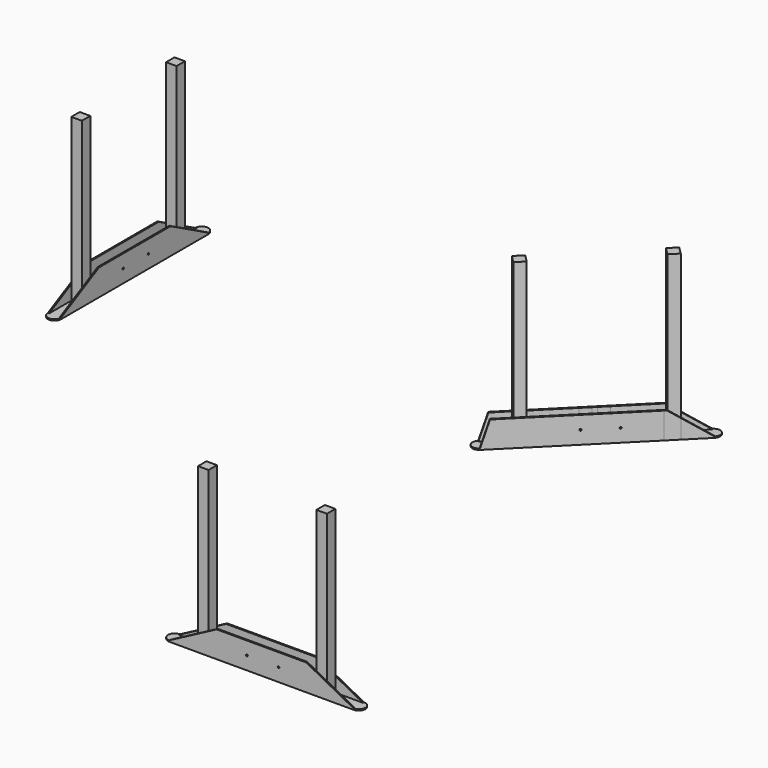
from build123d import *

# Parameters (mm, degrees)
F0_W           = 105
F0_H           = 40
F1_DEPTH       = 5
F0_W_2         = 40
F0_H_2         = 105
F2_DEPTH       = 620
F3_DEPTH       = 100
F4_T4_DEPTH    = 5
F4_T9_DEPTH    = 5
F4_T14_DEPTH   = 5
F4_T19_DEPTH   = 5
F4_2_T4_DEPTH  = 5
F4_2_T9_DEPTH  = 5
F4_2_T14_DEPTH = 5
F4_2_T19_DEPTH = 5
F6_T4_DEPTH    = 5
F6_T9_DEPTH    = 5
F7_SIZE2       = 94.99999
F7_SIZE        = 29.99999
F7_2_SIZE2     = 94.99999
F7_2_SIZE      = 29.99999
F10_R          = 3.25
F11_DEPTH      = 60
F12_R          = 3.25
F13_DEPTH      = 60
F14_R          = 3.25
F15_DEPTH      = 60


# Not quite as in the source:
# - a fillet or chamfer that OpenCascade refuses, or shapes differently, is made with other operations: its cross-section is extruded or revolved along the edge and cut away or added
# - two fillets or chamfers of one size are made in one step
# - a fillet or chamfer is up to 0.001 mm smaller than in the source, because OpenCascade refuses the exact size
# - a feature names something its author has since deleted; it is built from what else it names


with BuildPart() as f1:
    # F0 (on Top) → F1 (new body)
    with BuildSketch(Plane.XY):
        with BuildLine():
            ThreePointArc((811.153096903, -1265.8878414162), (836.153096903, -1240.8878414162), (811.153096903, -1215.8878414162))
            Line((811.153096903, -1215.8878414162), (811.153096903, -1220.8878414162))
            Line((811.153096903, -1220.8878414162), (811.153096903, -1260.8878414162))
            Line((811.153096903, -1260.8878414162), (811.153096903, -1265.8878414162))
        make_face()
        with Locations((758.653096903, -1240.8878414162)):
            Rectangle(F0_W, F0_H)
    extrude(amount=F1_DEPTH)



with BuildPart() as f1b:
    # F0 (on Top) → F1, piece 2 (new body)
    with BuildSketch(Plane.XY):
        with BuildLine():
            Line((111.153096903, -1220.8878414162), (111.153096903, -1215.8878414162))
            ThreePointArc((111.153096903, -1215.8878414162), (86.153096903, -1240.8878414162), (111.153096903, -1265.8878414162))
            Line((111.153096903, -1265.8878414162), (111.153096903, -1260.8878414162))
            Line((111.153096903, -1260.8878414162), (111.153096903, -1220.8878414162))
        make_face()
        with Locations((163.653096903, -1240.8878414162)):
            Rectangle(F0_W, F0_H)
    extrude(amount=F1_DEPTH)


with BuildPart() as f1c:
    # F0 (on Top) → F1, piece 3 (new body)
    with BuildSketch(Plane.XY):
        with BuildLine():
            Line((29.0142804433, 304.9314484107), (25.4787465374, 308.4669823167))
            ThreePointArc((25.4787465374, 308.4669823167), (25.4787465374, 273.1116432573), (60.8340855967, 273.1116432573))
            Line((60.8340855967, 273.1116432573), (57.2985516908, 276.6471771633))
            Line((57.2985516908, 276.6471771633), (29.0142804433, 304.9314484107))
        make_face()
        Polygon((99.724958562, 375.6421265294), (29.0142804433, 304.9314484107), (57.2985516908, 276.6471771633), (128.0092298094, 347.3578552819), align=None)
    extrude(amount=F1_DEPTH)



with BuildPart() as f1d:
    # F0 (on Top) → F1, piece 4 (new body)
    with BuildSketch(Plane.XY):
        with BuildLine():
            ThreePointArc((555.8088324273, 768.0863900879), (555.8088324273, 803.4417291473), (520.453493368, 803.4417291473))
            Line((520.453493368, 803.4417291473), (523.9890272739, 799.9061952413))
            Line((523.9890272739, 799.9061952413), (552.2732985214, 771.6219239939))
            Line((552.2732985214, 771.6219239939), (555.8088324273, 768.0863900879))
        make_face()
        Polygon((552.2732985214, 771.6219239939), (523.9890272739, 799.9061952413), (453.2783491552, 729.1955171227), (481.5626204027, 700.9112458752), align=None)
    extrude(amount=F1_DEPTH)


with BuildPart() as f1e:
    # F0 (on Top) → F1, piece 5 (new body)
    with BuildSketch(Plane.XY):
        with BuildLine():
            Line((-1479.9614127988, 152.1980424396), (-1484.9614127988, 152.1980424396))
            ThreePointArc((-1484.9614127988, 152.1980424396), (-1459.9614127988, 127.1980424396), (-1434.9614127988, 152.1980424396))
            Line((-1434.9614127988, 152.1980424396), (-1439.9614127988, 152.1980424396))
            Line((-1439.9614127988, 152.1980424396), (-1479.9614127988, 152.1980424396))
        make_face()
        Polygon((-1479.9614127988, 202.1980424396), (-1479.9614127988, 152.1980424396), (-1439.9614127988, 152.1980424396), (-1439.9614127988, 202.1980424396), (-1439.9614127988, 242.1980424396), (-1439.9614127988, 257.1980424396), (-1479.9614127988, 257.1980424396), (-1479.9614127988, 242.1980424396), align=None)
    extrude(amount=F1_DEPTH)



with BuildPart() as f1f:
    # F0 (on Top) → F1, piece 6 (new body)
    with BuildSketch(Plane.XY):
        with BuildLine():
            ThreePointArc((-1434.9614127988, 852.1980424396), (-1459.9614127988, 877.1980424396), (-1484.9614127988, 852.1980424396))
            Line((-1484.9614127988, 852.1980424396), (-1479.9614127988, 852.1980424396))
            Line((-1479.9614127988, 852.1980424396), (-1439.9614127988, 852.1980424396))
            Line((-1439.9614127988, 852.1980424396), (-1434.9614127988, 852.1980424396))
        make_face()
        with Locations((-1459.9614127988, 799.6980424396)):
            Rectangle(F0_W_2, F0_H_2)
    extrude(amount=F1_DEPTH)


with BuildPart() as f1g:
    # F0 (on Top) → F1, piece 7 (new body)
    with BuildSketch(Plane.XY):
        Polygon((331.153096903, -1220.8878414162), (256.153096903, -1220.8878414162), (256.153096903, -1260.8878414162), (331.153096903, -1260.8878414162), (421.153096903, -1260.8878414162), (511.153096903, -1260.8878414162), (591.153096903, -1260.8878414162), (666.153096903, -1260.8878414162), (666.153096903, -1220.8878414162), (591.153096903, -1220.8878414162), (511.153096903, -1220.8878414162), (421.153096903, -1220.8878414162), align=None)
    extrude(amount=F1_DEPTH)


with BuildPart() as f1h:
    # F0 (on Top) → F1, piece 8 (new body)
    with BuildSketch(Plane.XY):
        Polygon((-1439.9614127988, 707.1980424396), (-1479.9614127988, 707.1980424396), (-1479.9614127988, 542.1980424396), (-1479.9614127988, 502.1980424396), (-1479.9614127988, 297.1980424396), (-1439.9614127988, 297.1980424396), (-1439.9614127988, 502.1980424396), (-1439.9614127988, 542.1980424396), align=None)
    extrude(amount=F1_DEPTH)


with BuildPart() as f1i:
    # F0 (on Top) → F1, piece 9 (new body)
    with BuildSketch(Plane.XY):
        Polygon((241.1463147993, 517.0634827667), (128.0092298094, 403.9263977769), (156.2935010569, 375.6421265294), (269.4305860467, 488.7792115192), (297.7148572942, 517.0634827667), (304.7859251061, 524.1345505786), (333.0701963535, 552.418821826), (453.2783491552, 672.6269746277), (424.9940779078, 700.9112458752), (308.516985229, 584.4341531964), (280.2327139815, 556.149881949), (269.4305860467, 545.3477540142), align=None)
    extrude(amount=F1_DEPTH)


with BuildPart() as f1c_1:
    add(f1c.part)

    add(f1d.part)  # F2 merges F1d

    add(f1i.part)  # F2 merges F1i
    # F0 (on Top) → F2 (join)
    with BuildSketch(Plane.XY):
        Polygon((128.0092298094, 403.9263977769), (99.724958562, 375.6421265294), (128.0092298094, 347.3578552819), (156.2935010569, 375.6421265294), align=None)
        Polygon((481.5626204027, 700.9112458752), (453.2783491552, 729.1955171227), (424.9940779078, 700.9112458752), (453.2783491552, 672.6269746277), align=None)
    extrude(amount=F2_DEPTH)

    # F0 (on Top) → F3, piece 2 (join)
    with BuildSketch(Plane.XY):
        Polygon((392.9787465374, 675.9669823167), (43.156416067, 326.1446518463), (25.4787465374, 308.4669823167), (29.0142804433, 304.9314484107), (99.724958562, 375.6421265294), (128.0092298094, 403.9263977769), (241.1463147993, 517.0634827667), (269.4305860467, 545.3477540142), (280.2327139815, 556.149881949), (308.516985229, 584.4341531964), (424.9940779078, 700.9112458752), (453.2783491552, 729.1955171227), (523.9890272739, 799.9061952413), (520.453493368, 803.4417291473), (446.0117551264, 728.9999909057), (414.38747619, 697.3757119693), align=None)
        Polygon((57.2985516908, 276.6471771633), (60.8340855967, 273.1116432573), (78.5117551264, 290.789312787), (428.3340855967, 640.6116432573), (449.7428152493, 662.0203729099), (485.0981543086, 697.3757119693), (555.8088324273, 768.0863900879), (552.2732985214, 771.6219239939), (481.5626204027, 700.9112458752), (453.2783491552, 672.6269746277), (333.0701963535, 552.418821826), (304.7859251061, 524.1345505786), (297.7148572942, 517.0634827667), (269.4305860467, 488.7792115192), (156.2935010569, 375.6421265294), (128.0092298094, 347.3578552819), align=None)
    extrude(amount=F3_DEPTH)

    # F6: chamfer of 142 x 95 on 2 edges, made by hand


with BuildPart() as f1_1:
    add(f1.part)

    add(f1b.part)  # F2#2 merges F1b

    add(f1g.part)  # F2#2 merges F1g
    # F0 (on Top) → F2, piece 2 (join)
    with BuildSketch(Plane.XY):
        with Locations((686.153096903, -1240.8878414162)):
            Rectangle(F0_W_2, F0_H)
        with Locations((236.153096903, -1240.8878414162)):
            Rectangle(F0_W_2, F0_H)
    extrude(amount=F2_DEPTH)

    # F0 (on Top) → F3, piece 3 (join)
    with BuildSketch(Plane.XY):
        Polygon((811.153096903, -1215.8878414162), (111.153096903, -1215.8878414162), (111.153096903, -1220.8878414162), (216.153096903, -1220.8878414162), (256.153096903, -1220.8878414162), (331.153096903, -1220.8878414162), (421.153096903, -1220.8878414162), (511.153096903, -1220.8878414162), (591.153096903, -1220.8878414162), (666.153096903, -1220.8878414162), (706.153096903, -1220.8878414162), (811.153096903, -1220.8878414162), align=None)
        Polygon((111.153096903, -1260.8878414162), (111.153096903, -1265.8878414162), (811.153096903, -1265.8878414162), (811.153096903, -1260.8878414162), (706.153096903, -1260.8878414162), (666.153096903, -1260.8878414162), (591.153096903, -1260.8878414162), (511.153096903, -1260.8878414162), (421.153096903, -1260.8878414162), (331.153096903, -1260.8878414162), (256.153096903, -1260.8878414162), (216.153096903, -1260.8878414162), align=None)
    extrude(amount=F3_DEPTH)

    # F4: chamfer of 180 x 95 on 4 edges, made by hand


with BuildPart() as f1e_1:
    add(f1e.part)

    add(f1f.part)  # F2#3 merges F1f

    add(f1h.part)  # F2#3 merges F1h
    # F0 (on Top) → F2, piece 3 (join)
    with BuildSketch(Plane.XY):
        with Locations((-1459.9614127988, 727.1980424396)):
            Rectangle(F0_W_2, F0_H)
        with Locations((-1459.9614127988, 277.1980424396)):
            Rectangle(F0_W_2, F0_H)
    extrude(amount=F2_DEPTH)

    # F0 (on Top) → F3 (join)
    with BuildSketch(Plane.XY):
        Polygon((-1484.9614127988, 852.1980424396), (-1484.9614127988, 152.1980424396), (-1479.9614127988, 152.1980424396), (-1479.9614127988, 202.1980424396), (-1479.9614127988, 242.1980424396), (-1479.9614127988, 257.1980424396), (-1479.9614127988, 297.1980424396), (-1479.9614127988, 502.1980424396), (-1479.9614127988, 542.1980424396), (-1479.9614127988, 707.1980424396), (-1479.9614127988, 747.1980424396), (-1479.9614127988, 852.1980424396), align=None)
        Polygon((-1439.9614127988, 152.1980424396), (-1434.9614127988, 152.1980424396), (-1434.9614127988, 852.1980424396), (-1439.9614127988, 852.1980424396), (-1439.9614127988, 747.1980424396), (-1439.9614127988, 707.1980424396), (-1439.9614127988, 542.1980424396), (-1439.9614127988, 502.1980424396), (-1439.9614127988, 297.1980424396), (-1439.9614127988, 257.1980424396), (-1439.9614127988, 242.1980424396), (-1439.9614127988, 202.1980424396), align=None)
    extrude(amount=F3_DEPTH)

    # F4#2: chamfer of 180 x 95 on 4 edges, made by hand


with BuildPart() as f4_tool2:
    # F4_s3 → F4_t4 (new body)
    with BuildSketch(Plane.XZ.offset(1260.8878414162)):
        with BuildLine():
            Line((297.5206671235, 103.3606620608), (104.7855266825, 1.6393379392))
            Line((104.7855266825, 1.6393379392), (101.1855266825, 1.6393379392))
            ThreePointArc((101.1855266825, 1.6393379392), (107.553096903, 50.8196689696), (107.553096903, 100))
            Line((107.553096903, 100), (111.153096903, 103.6))
            ThreePointArc((111.153096903, 103.6), (204.3368820132, 103.6), (297.5206671235, 106.9606620608))
            Line((297.5206671235, 106.9606620608), (297.5206671235, 103.3606620608))
        make_face()
    extrude(amount=F4_T4_DEPTH)

    split(bisect_by=Plane.XY.offset(5), keep=Keep.TOP)


with BuildPart() as f1_2:
    add(f1_1.part)

    # F4_t1: cut F4_tool2
    add(f4_tool2.part, mode=Mode.SUBTRACT)


with BuildPart() as f4_tool7:
    # F4_s8 → F4_t9 (new body)
    with BuildSketch(Plane.XZ.offset(1215.8878414162)):
        with BuildLine():
            Line((297.5206671235, 103.3606620608), (104.7855266825, 1.6393379392))
            Line((104.7855266825, 1.6393379392), (101.1855266825, 1.6393379392))
            ThreePointArc((101.1855266825, 1.6393379392), (107.553096903, 50.8196689696), (107.553096903, 100))
            Line((107.553096903, 100), (111.153096903, 103.6))
            ThreePointArc((111.153096903, 103.6), (204.3368820132, 103.6), (297.5206671235, 106.9606620608))
            Line((297.5206671235, 106.9606620608), (297.5206671235, 103.3606620608))
        make_face()
    extrude(amount=F4_T9_DEPTH)

    split(bisect_by=Plane.XY.offset(5), keep=Keep.TOP)


with BuildPart() as f1_3:
    add(f1_2.part)

    # F4_t6: cut F4_tool7
    add(f4_tool7.part, mode=Mode.SUBTRACT)


with BuildPart() as f4_tool12:
    # F4_s13 → F4_t14 (new body)
    with BuildSketch(Plane.XZ.offset(1265.8878414162)):
        with BuildLine():
            Line((624.7855266825, 103.3606620608), (817.5206671235, 1.6393379392))
            Line((817.5206671235, 1.6393379392), (821.1206671235, 1.6393379392))
            ThreePointArc((821.1206671235, 1.6393379392), (814.753096903, 50.8196689696), (814.753096903, 100))
            Line((814.753096903, 100), (811.153096903, 103.6))
            ThreePointArc((811.153096903, 103.6), (717.9693117927, 103.6), (624.7855266825, 106.9606620608))
            Line((624.7855266825, 106.9606620608), (624.7855266825, 103.3606620608))
        make_face()
    extrude(amount=-F4_T14_DEPTH)

    split(bisect_by=Plane.XY.offset(5), keep=Keep.TOP)


with BuildPart() as f1_4:
    add(f1_3.part)

    # F4_t11: cut F4_tool12
    add(f4_tool12.part, mode=Mode.SUBTRACT)


with BuildPart() as f4_tool17:
    # F4_s18 → F4_t19 (new body)
    with BuildSketch(Plane.XZ.offset(1220.8878414162)):
        with BuildLine():
            Line((624.7855266825, 103.3606620608), (817.5206671235, 1.6393379392))
            Line((817.5206671235, 1.6393379392), (821.1206671235, 1.6393379392))
            ThreePointArc((821.1206671235, 1.6393379392), (814.753096903, 50.8196689696), (814.753096903, 100))
            Line((814.753096903, 100), (811.153096903, 103.6))
            ThreePointArc((811.153096903, 103.6), (717.9693117927, 103.6), (624.7855266825, 106.9606620608))
            Line((624.7855266825, 106.9606620608), (624.7855266825, 103.3606620608))
        make_face()
    extrude(amount=-F4_T19_DEPTH)

    split(bisect_by=Plane.XY.offset(5), keep=Keep.TOP)


with BuildPart() as f1_5:
    add(f1_4.part)

    # F4_t16: cut F4_tool17
    add(f4_tool17.part, mode=Mode.SUBTRACT)

    # F9: union 

    # F10 (on face) → F11 (cut)
    with BuildSketch(Plane.XZ.offset(1265.8878414162)):
        with Locations((406.153096903, 50)):
            Circle(F10_R)
        with Locations((526.153096903, 50)):
            Circle(F10_R)
    extrude(amount=-F11_DEPTH, mode=Mode.SUBTRACT)


with BuildPart() as f4_2_tool2:
    # F4_2_s3 → F4_2_t4 (new body)
    with BuildSketch(Plane.YZ.offset(-1484.9614127988)):
        with BuildLine():
            Line((338.5656126601, 103.3606620608), (145.8304722191, 1.6393379392))
            Line((145.8304722191, 1.6393379392), (142.2304722191, 1.6393379392))
            ThreePointArc((142.2304722191, 1.6393379392), (148.5980424396, 50.8196689696), (148.5980424396, 100))
            Line((148.5980424396, 100), (152.1980424396, 103.6))
            ThreePointArc((152.1980424396, 103.6), (245.3818275499, 103.6), (338.5656126601, 106.9606620608))
            Line((338.5656126601, 106.9606620608), (338.5656126601, 103.3606620608))
        make_face()
    extrude(amount=F4_2_T4_DEPTH)

    split(bisect_by=Plane.XY.offset(5), keep=Keep.TOP)


with BuildPart() as f1e_2:
    add(f1e_1.part)

    # F4_2_t1: cut F4_2_tool2
    add(f4_2_tool2.part, mode=Mode.SUBTRACT)


with BuildPart() as f4_2_tool7:
    # F4_2_s8 → F4_2_t9 (new body)
    with BuildSketch(Plane.YZ.offset(-1479.9614127988)):
        with BuildLine():
            Line((665.8304722191, 103.3606620608), (858.5656126601, 1.6393379392))
            Line((858.5656126601, 1.6393379392), (862.1656126601, 1.6393379392))
            ThreePointArc((862.1656126601, 1.6393379392), (855.7980424396, 50.8196689696), (855.7980424396, 100))
            Line((855.7980424396, 100), (852.1980424396, 103.6))
            ThreePointArc((852.1980424396, 103.6), (759.0142573294, 103.6), (665.8304722191, 106.9606620608))
            Line((665.8304722191, 106.9606620608), (665.8304722191, 103.3606620608))
        make_face()
    extrude(amount=-F4_2_T9_DEPTH)

    split(bisect_by=Plane.XY.offset(5), keep=Keep.TOP)


with BuildPart() as f1e_3:
    add(f1e_2.part)

    # F4_2_t6: cut F4_2_tool7
    add(f4_2_tool7.part, mode=Mode.SUBTRACT)


with BuildPart() as f4_2_tool12:
    # F4_2_s13 → F4_2_t14 (new body)
    with BuildSketch(Plane.YZ.offset(-1439.9614127988)):
        with BuildLine():
            Line((338.5656126601, 103.3606620608), (145.8304722191, 1.6393379392))
            Line((145.8304722191, 1.6393379392), (142.2304722191, 1.6393379392))
            ThreePointArc((142.2304722191, 1.6393379392), (148.5980424396, 50.8196689696), (148.5980424396, 100))
            Line((148.5980424396, 100), (152.1980424396, 103.6))
            ThreePointArc((152.1980424396, 103.6), (245.3818275499, 103.6), (338.5656126601, 106.9606620608))
            Line((338.5656126601, 106.9606620608), (338.5656126601, 103.3606620608))
        make_face()
    extrude(amount=F4_2_T14_DEPTH)

    split(bisect_by=Plane.XY.offset(5), keep=Keep.TOP)


with BuildPart() as f1e_4:
    add(f1e_3.part)

    # F4_2_t11: cut F4_2_tool12
    add(f4_2_tool12.part, mode=Mode.SUBTRACT)


with BuildPart() as f4_2_tool17:
    # F4_2_s18 → F4_2_t19 (new body)
    with BuildSketch(Plane.YZ.offset(-1434.9614127988)):
        with BuildLine():
            Line((665.8304722191, 103.3606620608), (858.5656126601, 1.6393379392))
            Line((858.5656126601, 1.6393379392), (862.1656126601, 1.6393379392))
            ThreePointArc((862.1656126601, 1.6393379392), (855.7980424396, 50.8196689696), (855.7980424396, 100))
            Line((855.7980424396, 100), (852.1980424396, 103.6))
            ThreePointArc((852.1980424396, 103.6), (759.0142573294, 103.6), (665.8304722191, 106.9606620608))
            Line((665.8304722191, 106.9606620608), (665.8304722191, 103.3606620608))
        make_face()
    extrude(amount=-F4_2_T19_DEPTH)

    split(bisect_by=Plane.XY.offset(5), keep=Keep.TOP)


with BuildPart() as f1e_5:
    add(f1e_4.part)

    # F4_2_t16: cut F4_2_tool17
    add(f4_2_tool17.part, mode=Mode.SUBTRACT)

    # F8: union 

    # F14 (on face) → F15 (cut)
    with BuildSketch(Plane(origin=(-1484.9614127988, 0, 0), x_dir=(0, -1, 0), z_dir=(-1, 0, 0))):
        with Locations((-567.1980424396, 50)):
            Circle(F14_R)
        with Locations((-447.1980424396, 50)):
            Circle(F14_R)
    extrude(amount=-F15_DEPTH, mode=Mode.SUBTRACT)


with BuildPart() as f6_tool2:
    # F6_s3 → F6_t4 (new body)
    with BuildSketch(Plane(origin=(-106.1387788303, 106.1387788303, 0), x_dir=(0, 0, 1), z_dir=(-0.7071067812, 0.7071067812, 0))):
        with BuildLine():
            Line((103.1583651049, 789.4143647378), (1.8416348951, 940.8562141041))
            Line((1.8416348951, 940.8562141041), (1.8416348951, 943.6962141041))
            ThreePointArc((1.8416348951, 943.6962141041), (50.9208174475, 938.975289421), (100, 938.975289421))
            Line((100, 938.975289421), (102.84, 936.135289421))
            ThreePointArc((102.84, 936.135289421), (102.84, 862.7748270794), (105.9983651049, 789.4143647378))
            Line((105.9983651049, 789.4143647378), (103.1583651049, 789.4143647378))
        make_face()
    extrude(amount=F6_T4_DEPTH)

    split(bisect_by=Plane.XY.offset(5), keep=Keep.TOP)


with BuildPart() as f1c_2:
    add(f1c_1.part)

    # F6_t1: cut F6_tool2
    add(f6_tool2.part, mode=Mode.SUBTRACT)


with BuildPart() as f6_tool7:
    # F6_s8 → F6_t9 (new body)
    with BuildSketch(Plane(origin=(-137.9585839837, 137.9585839837, 0), x_dir=(0, 0, 1), z_dir=(-0.7071067812, 0.7071067812, 0))):
        with BuildLine():
            Line((103.1583651049, 789.4143647378), (1.8416348951, 940.8562141041))
            Line((1.8416348951, 940.8562141041), (1.8416348951, 943.6962141041))
            ThreePointArc((1.8416348951, 943.6962141041), (50.9208174475, 938.975289421), (100, 938.975289421))
            Line((100, 938.975289421), (102.84, 936.135289421))
            ThreePointArc((102.84, 936.135289421), (102.84, 862.7748270794), (105.9983651049, 789.4143647378))
            Line((105.9983651049, 789.4143647378), (103.1583651049, 789.4143647378))
        make_face()
    extrude(amount=F6_T9_DEPTH)

    split(bisect_by=Plane.XY.offset(5), keep=Keep.TOP)


with BuildPart() as f1c_3:
    add(f1c_2.part)

    # F6_t6: cut F6_tool7
    add(f6_tool7.part, mode=Mode.SUBTRACT)

    # F7 (size 30 and 95 in the source; OpenCascade refuses exactly that, so slightly less here)
    f7_edges = [f1c_3.edges().sort_by_distance(p)[0] for p in [
        (59.066319, 274.87941, 100),
    ]]
    f7_side = f1c_3.faces().sort_by_distance((256.349111, 472.162202, 100))[0]
    chamfer(f7_edges, length=F7_SIZE, length2=F7_SIZE2, reference=f7_side)

    # F7#2 (size 30 and 95 in the source; OpenCascade refuses exactly that, so slightly less here)
    f7_2_edges = [f1c_3.edges().sort_by_distance(p)[0] for p in [
        (27.246513, 306.699215, 100),
    ]]
    f7_2_side = f1c_3.faces().sort_by_distance((224.529305, 503.982007, 100))[0]
    chamfer(f7_2_edges, length=F7_2_SIZE, length2=F7_2_SIZE2, reference=f7_2_side)

    # F12 (on face) → F13 (cut)
    with BuildSketch(Plane(origin=(-106.1387788303, 106.1387788303, 0), x_dir=(0.7071067812, 0.7071067812, 0), z_dir=(0.7071067812, -0.7071067812, 0))):
        with Locations((536.135289421, 50)):
            Circle(F12_R)
        with Locations((656.135289421, 50)):
            Circle(F12_R)
    extrude(amount=-F13_DEPTH, mode=Mode.SUBTRACT)


solid = Compound([f1_5.part, f1e_5.part, f1c_3.part])
